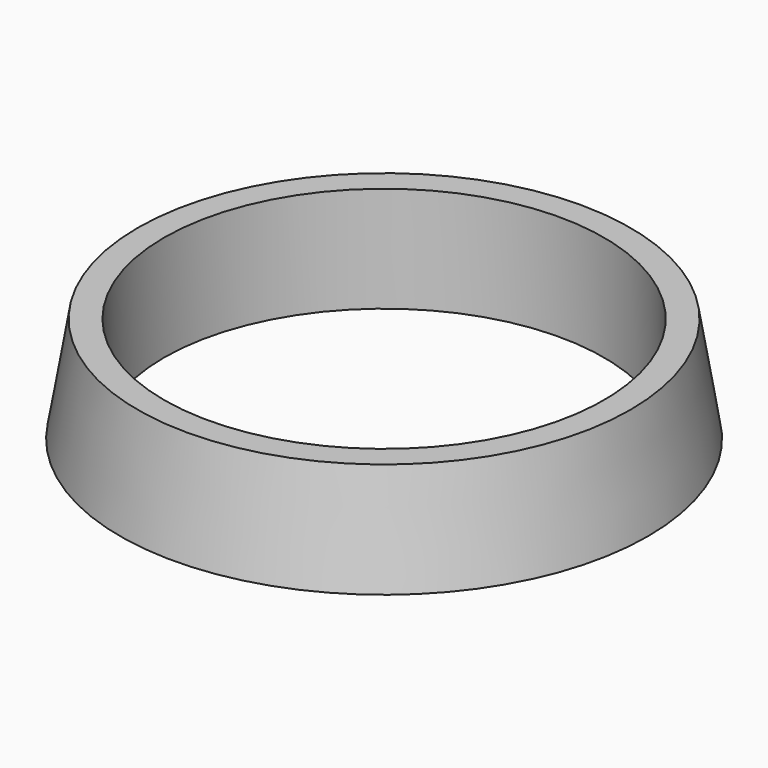
from build123d import *

# Parameters (mm, degrees)
F0_R     = 1.5
F1_DEPTH = 0.6
F2_D     = 2.5
F3_SIZE2 = 0.59999
F3_SIZE  = 0.09999


# Not quite as in the source:
# - a fillet or chamfer is up to 0.001 mm smaller than in the source, because OpenCascade refuses the exact size


with BuildPart() as f1:
    # F0 (on Top) → F1 (new body)
    with BuildSketch(Plane.XY):
        Circle(F0_R)
    extrude(amount=F1_DEPTH)

    # F2 (through all)
    with Locations(Plane(origin=(0, 0, 0), x_dir=(1, 0, 0), z_dir=(0, 0, -1))):
        with Locations((0, 0)):
            Hole(F2_D / 2)

    # F3 (size 0.1 and 0.6 in the source; OpenCascade refuses exactly that, so slightly less here)
    f3_edges = [f1.edges().sort_by_distance(p)[0] for p in [
        (-1.5, 0, 0.6),
    ]]
    f3_side = f1.faces().sort_by_distance((-1.457574, 0, 0.6))[0]
    chamfer(f3_edges, length=F3_SIZE, length2=F3_SIZE2, reference=f3_side)


solid = f1.part
